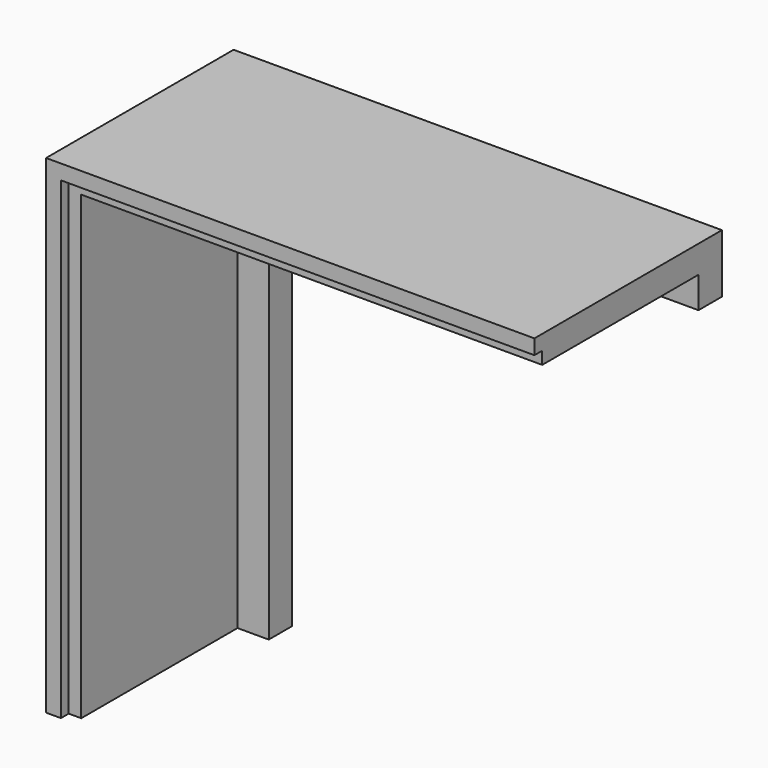
from build123d import *

# Parameters (mm, degrees)
F1_DEPTH = 76.2
F2_W     = 153.924
F2_H     = 153.924
F3_DEPTH = 3.175
F4_W     = 149.86
F4_H     = 149.86
F5_DEPTH = 63.5


# Not quite as in the source:
# - a feature names something its author has since deleted; it is built from what else it names


with BuildPart() as f1:
    # F0 (on Front) → F1 (new body)
    with BuildSketch(Plane.XZ):
        Polygon((0, 139.7), (0, 158.75), (-158.75, 158.75), (-158.75, 0), (-139.7, 0), (-139.7, 139.7), align=None)
    extrude(amount=F1_DEPTH)

    # F2 (on face) → F3 (cut)
    with BuildSketch(Plane.XZ.offset(76.2)):
        with Locations((-76.962, 76.962)):
            Rectangle(F2_W, F2_H)
    extrude(amount=-F3_DEPTH, mode=Mode.SUBTRACT)

    # F4 (on face) → F5 (cut)
    with BuildSketch(Plane.XZ.offset(73.025)):
        with Locations((-74.93, 74.93)):
            Rectangle(F4_W, F4_H)
    extrude(amount=-F5_DEPTH, mode=Mode.SUBTRACT)


solid = f1.part
